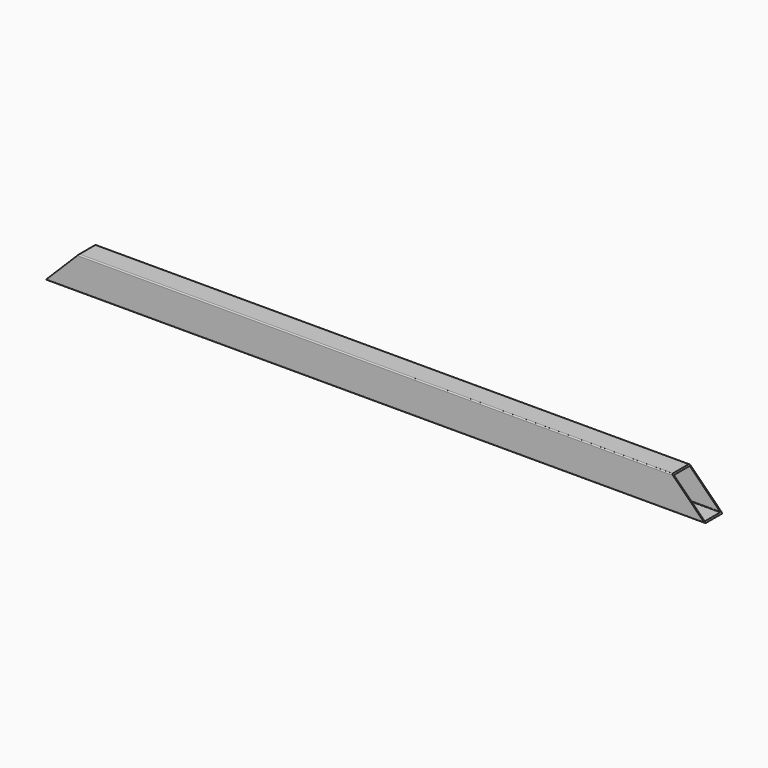
from build123d import *

# Parameters (mm, degrees)
F1_DEPTH      = 600
F1_DEPTH_BACK = 600
F3_DEPTH      = 25
F3_DEPTH_BACK = 25


with BuildPart() as f1:
    # F0 (on Right) → F1 (new body, two sides)
    with BuildSketch(Plane.YZ) as f1_sk:
        with BuildLine():
            ThreePointArc((-20, -28), (-19.4142135624, -29.4142135624), (-18, -30))
            Line((-18, -30), (18, -30))
            ThreePointArc((18, -30), (19.4142135624, -29.4142135624), (20, -28))
            Line((20, -28), (20, 28))
            ThreePointArc((20, 28), (19.4142135624, 29.4142135624), (18, 30))
            Line((18, 30), (-18, 30))
            ThreePointArc((-18, 30), (-19.4142135624, 29.4142135624), (-20, 28))
            Line((-20, 28), (-20, -28))
        make_face()
        with BuildLine():
            Line((17, -28), (-17, -28))
            ThreePointArc((-17, -28), (-17.7071067812, -27.7071067812), (-18, -27))
            Line((-18, -27), (-18, 27))
            ThreePointArc((-18, 27), (-17.7071067812, 27.7071067812), (-17, 28))
            Line((-17, 28), (17, 28))
            ThreePointArc((17, 28), (17.7071067812, 27.7071067812), (18, 27))
            Line((18, 27), (18, -27))
            ThreePointArc((18, -27), (17.7071067812, -27.7071067812), (17, -28))
        make_face(mode=Mode.SUBTRACT)
    extrude(amount=F1_DEPTH)
    extrude(f1_sk.sketch, amount=-F1_DEPTH_BACK)

    # F2 (on Front) → F3 (cut, two sides)
    with BuildSketch(Plane.XZ) as f3_sk:
        Polygon((-600, 30), (-600, -30), (-540, 30), align=None)
        Polygon((540, 30), (600, -30), (600, 30), align=None)
    extrude(amount=-F3_DEPTH, mode=Mode.SUBTRACT)
    extrude(f3_sk.sketch, amount=F3_DEPTH_BACK, mode=Mode.SUBTRACT)


solid = f1.part
